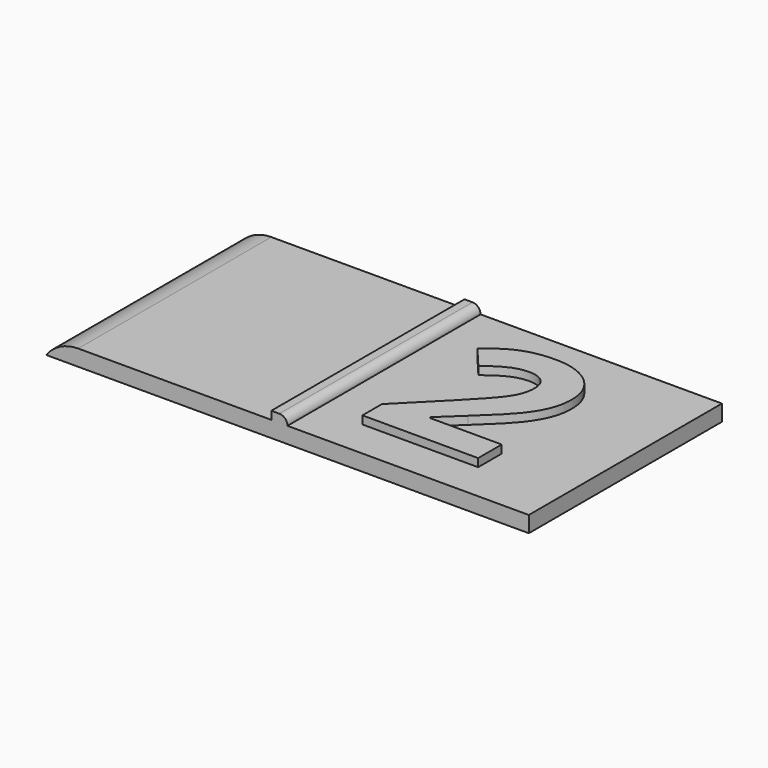
from build123d import *

# Parameters (mm, degrees)
F0_W         = 60
F0_H         = 30
F1_DEPTH     = 2
F2_W         = 2
F2_H         = 30
F3_DEPTH     = 1
F4_R         = 0.99999
F5_TEXT_SIZE = 28.8201948731
F6_DEPTH     = 1
F7_T1_DEPTH  = 50


# Not quite as in the source:
# - a fillet or chamfer that OpenCascade refuses, or shapes differently, is made with other operations: its cross-section is extruded or revolved along the edge and cut away or added
# - a fillet or chamfer is up to 0.001 mm smaller than in the source, because OpenCascade refuses the exact size
# - Text() gives the source's letters only with a copy of the font that has no kerning and outlines rounded to 1/6400 em; it was checked with that copy


with BuildPart() as f1:
    # F0 (on Top) → F1 (new body)
    with BuildSketch(Plane.XY):
        with Locations((30, 15)):
            Rectangle(F0_W, F0_H)
    extrude(amount=F1_DEPTH)

    # F2 (on face) → F3 (join)
    with BuildSketch(Plane.XY.offset(2)):
        with Locations((29, 15)):
            Rectangle(F2_W, F2_H)
    extrude(amount=F3_DEPTH)

    # F4 (radius 1 in the source; OpenCascade refuses exactly that, so slightly less here)
    f4_edges = [f1.edges().sort_by_distance(p)[0] for p in [
        (30, 15, 3),
    ]]
    fillet(f4_edges, radius=F4_R)

    # F5 (on face) → F6 (join)
    with BuildSketch(Plane.XY.offset(2)):
        with Locations((34.3574509025, 4.7624194995)):
            Text('2', F5_TEXT_SIZE, font='Open Sans', font_style=FontStyle.BOLD, text_align=(TextAlign.LEFT, TextAlign.BOTTOM))
    extrude(amount=F6_DEPTH)

    # F7: fillet of radius 5 on 1 edges, made by hand

    # F7_s2 → F7_t1 (cut)
    with BuildSketch(Plane.XZ.offset(-40)):
        with BuildLine():
            ThreePointArc((4, 2), (1.7639320225, 1.472135955), (0, 0))
            Line((0, 0), (0, 2))
            Line((0, 2), (4, 2))
        make_face()
    extrude(amount=F7_T1_DEPTH, mode=Mode.SUBTRACT)


solid = f1.part
